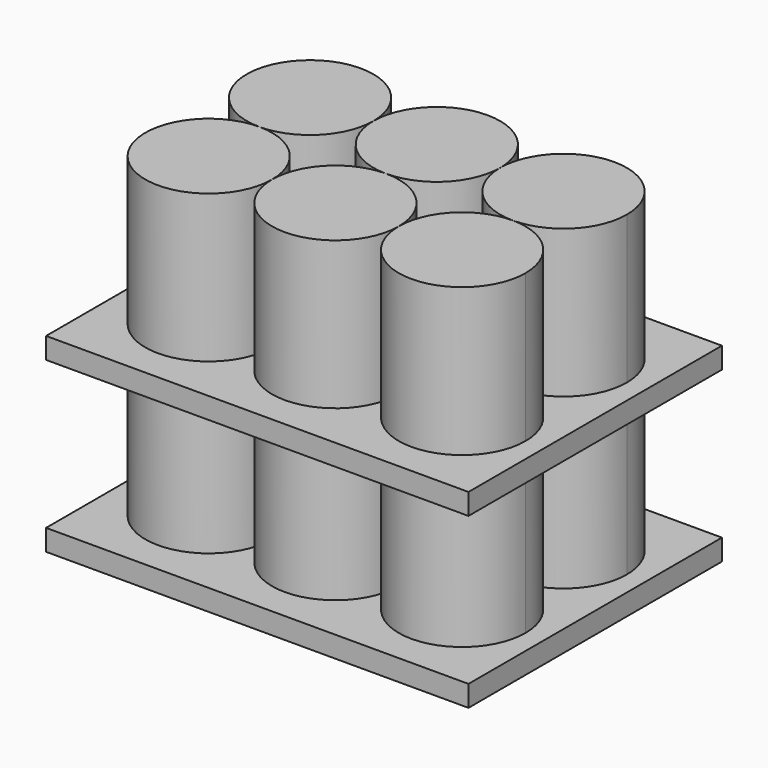
from build123d import *

# Parameters (mm, degrees)
F1_DEPTH = 76.2
F2_W     = 101.6
F2_H     = 5.08
F3_DEPTH = 38.1
F2_H_2   = 5.0807343126


# Not quite as in the source:
# - a feature names something its author has since deleted; it is built from what else it names


with BuildPart() as f1:
    # F0 (on Top) → F1 (new body)
    with BuildSketch(Plane.XY):
        with BuildLine():
            ThreePointArc((-29.9686177893, -0.0085821988), (-40.7449251346, -26.0248895441), (-14.7286177893, -15.2485821988))
            ThreePointArc((-14.7286177893, -15.2485821988), (-19.192310444, -4.4722748535), (-29.9686177893, -0.0085821988))
        make_face()
    extrude(amount=F1_DEPTH)


with BuildPart() as f1b:
    # F0 (on Top) → F1, piece 2 (new body)
    with BuildSketch(Plane.XY):
        with BuildLine():
            ThreePointArc((0.5113822094, -0.0085821988), (-10.264925135, -4.472274854), (-14.7286177893, -15.2485821988))
            ThreePointArc((-14.7286177893, -15.2485821988), (0.5113822107, -30.4885821988), (15.7513822107, -15.2485821988))
            ThreePointArc((15.7513822107, -15.2485821988), (11.2876895555, -4.4722748531), (0.5113822094, -0.0085821988))
        make_face()
    extrude(amount=F1_DEPTH)


with BuildPart() as f1c:
    # F0 (on Top) → F1, piece 3 (new body)
    with BuildSketch(Plane.XY):
        with BuildLine():
            ThreePointArc((-14.7286177893, 15.2314178012), (-40.7449251346, 26.0077251465), (-29.9686177893, -0.0085821988))
            ThreePointArc((-29.9686177893, -0.0085821988), (-19.192310444, 4.4551104559), (-14.7286177893, 15.2314178012))
        make_face()
    extrude(amount=F1_DEPTH)


with BuildPart() as f1d:
    # F0 (on Top) → F1, piece 4 (new body)
    with BuildSketch(Plane.XY):
        with BuildLine():
            ThreePointArc((30.9913822354, -0.0085821988), (20.2150748742, -4.4722748448), (15.7513822107, -15.2485821988))
            ThreePointArc((15.7513822107, -15.2485821988), (30.9913822107, -30.4885821988), (46.2313822107, -15.2485821988))
            ThreePointArc((46.2313822107, -15.2485821988), (41.7676895647, -4.4722748623), (30.9913822354, -0.0085821988))
        make_face()
    extrude(amount=F1_DEPTH)


with BuildPart() as f1e:
    # F0 (on Top) → F1, piece 5 (new body)
    with BuildSketch(Plane.XY):
        with BuildLine():
            ThreePointArc((-14.7286177893, 15.2314178012), (-10.264925135, 4.4551104564), (0.5113822094, -0.0085821988))
            ThreePointArc((0.5113822094, -0.0085821988), (11.2876895555, 4.4551104555), (15.7513822107, 15.2314178012))
            ThreePointArc((15.7513822107, 15.2314178012), (0.5113822107, 30.4714178012), (-14.7286177893, 15.2314178012))
        make_face()
    extrude(amount=F1_DEPTH)


with BuildPart() as f1f:
    # F0 (on Top) → F1, piece 6 (new body)
    with BuildSketch(Plane.XY):
        with BuildLine():
            ThreePointArc((15.7513822107, 15.2314178012), (20.2150748742, 4.4551104472), (30.9913822354, -0.0085821988))
            ThreePointArc((30.9913822354, -0.0085821988), (41.7676895647, 4.4551104647), (46.2313822107, 15.2314178012))
            ThreePointArc((46.2313822107, 15.2314178012), (30.9913822107, 30.4714178012), (15.7513822107, 15.2314178012))
        make_face()
    extrude(amount=F1_DEPTH)


with BuildPart() as f3:
    # F2 (on Front) → F3 (new body, symmetric)
    with BuildSketch(Plane.XZ):
        with Locations((0, -2.54)):
            Rectangle(F2_W, F2_H)
    extrude(amount=F3_DEPTH, both=True)


with BuildPart() as f3b:
    # F2 (on Front) → F3, piece 2 (new body, symmetric)
    with BuildSketch(Plane.XZ):
        with Locations((0, 38.1003671563)):
            Rectangle(F2_W, F2_H_2)
    extrude(amount=F3_DEPTH, both=True)


solid = Compound([f1.part, f1b.part, f1c.part, f1d.part, f1e.part, f1f.part, f3.part, f3b.part])
